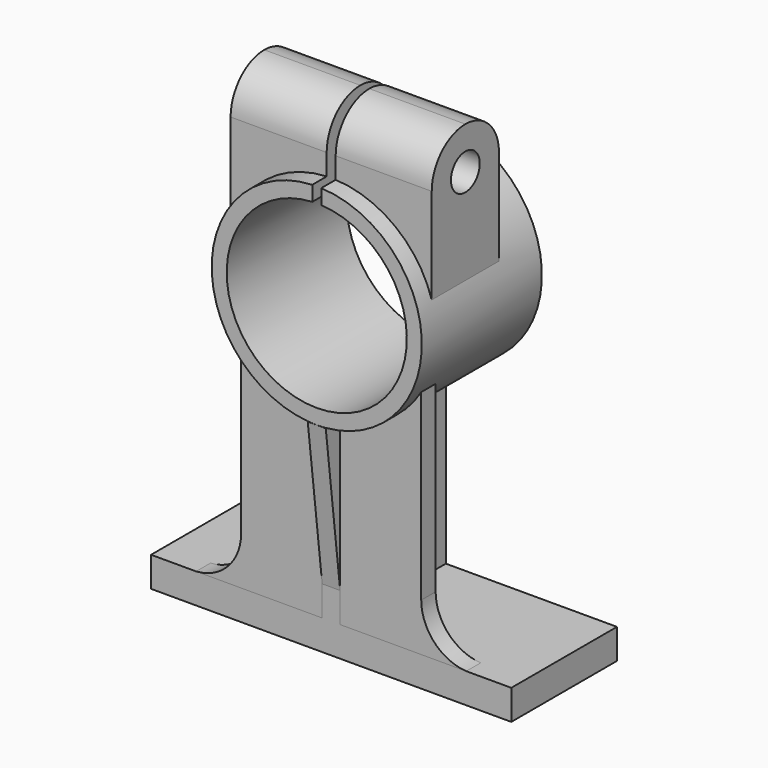
from build123d import *

# Parameters (mm, degrees)
F1_DEPTH = 6
F2_DEPTH = 44
F0_W     = 6
F0_H     = 10
F3_DEPTH = 6
F4_DEPTH = 28
F6_DEPTH = 93.501
F7_DEPTH = 93.501


with BuildPart() as f1:
    # F0 (on Front) → F1 (new body)
    with BuildSketch(Plane.XZ):
        with BuildLine():
            ThreePointArc((-33.5, 10.1365674664), (-34.7328343847, -4.3162733471), (-30, -18.0277563773))
            ThreePointArc((-30, -18.0277563773), (-18.5249919592, -29.695532878), (-3, -34.8711915483))
            ThreePointArc((-3, -34.8711915483), (-1.5013819904, -34.9677830598), (1.54e-08, -35))
            ThreePointArc((1.54e-08, -35), (1.5013820058, -34.9677830592), (3, -34.8711915483))
            ThreePointArc((3, -34.8711915483), (18.5249919592, -29.695532878), (30, -18.0277563773))
            ThreePointArc((30, -18.0277563773), (34.7328343847, -4.3162733471), (33.5, 10.1365674664))
            ThreePointArc((33.5, 10.1365674664), (21.4568882491, 27.6514366113), (1.5, 34.9678423698))
            Line((1.5, 34.9678423698), (1.5, 29.9624765332))
            ThreePointArc((1.5, 29.9624765332), (0, -30), (-1.5, 29.9624765332))
            Line((-1.5, 29.9624765332), (-1.5, 34.9678423698))
            ThreePointArc((-1.5, 34.9678423698), (-21.4568882491, 27.6514366113), (-33.5, 10.1365674664))
        make_face()
    extrude(amount=F1_DEPTH)

    # F0 (on Front) → F2 (join)
    with BuildSketch(Plane.XZ):
        with BuildLine():
            ThreePointArc((-33.5, 10.1365674664), (-34.7328343847, -4.3162733471), (-30, -18.0277563773))
            ThreePointArc((-30, -18.0277563773), (-18.5249919592, -29.695532878), (-3, -34.8711915483))
            ThreePointArc((-3, -34.8711915483), (-1.5013819904, -34.9677830598), (1.54e-08, -35))
            ThreePointArc((1.54e-08, -35), (1.5013820058, -34.9677830592), (3, -34.8711915483))
            ThreePointArc((3, -34.8711915483), (18.5249919592, -29.695532878), (30, -18.0277563773))
            ThreePointArc((30, -18.0277563773), (34.7328343847, -4.3162733471), (33.5, 10.1365674664))
            ThreePointArc((33.5, 10.1365674664), (21.4568882491, 27.6514366113), (1.5, 34.9678423698))
            Line((1.5, 34.9678423698), (1.5, 29.9624765332))
            ThreePointArc((1.5, 29.9624765332), (0, -30), (-1.5, 29.9624765332))
            Line((-1.5, 29.9624765332), (-1.5, 34.9678423698))
            ThreePointArc((-1.5, 34.9678423698), (-21.4568882491, 27.6514366113), (-33.5, 10.1365674664))
        make_face()
    extrude(amount=-F2_DEPTH)

    # F0 (on Front) → F3 (join)
    with BuildSketch(Plane.XZ):
        with BuildLine():
            Line((-30, -18.0277563773), (-30, -35))
            Line((-30, -35), (-3, -35))
            Line((-3, -35), (-3, -34.8711915483))
            ThreePointArc((-3, -34.8711915483), (-18.5249919592, -29.695532878), (-30, -18.0277563773))
        make_face()
        with BuildLine():
            Line((3, -34.8711915483), (3, -35))
            Line((3, -35), (30, -35))
            Line((30, -35), (30, -18.0277563773))
            ThreePointArc((30, -18.0277563773), (18.5249919592, -29.695532878), (3, -34.8711915483))
        make_face()
        with BuildLine():
            Line((-30, -95), (-30, -79.0312805773))
            ThreePointArc((-30, -79.0312805773), (-34.3380962103, -89.9857317274), (-45, -95))
            Line((-45, -95), (-30, -95))
        make_face()
        with BuildLine():
            ThreePointArc((45, -95), (34.3380962103, -89.9857317274), (30, -79.0312805773))
            Line((30, -79.0312805773), (30, -95))
            Line((30, -95), (45, -95))
        make_face()
        Polygon((-3, -35), (-30, -35), (-30, -79.0312805773), (-30, -95), (-3, -95), (-3, -85), align=None)
        Polygon((30, -35), (3, -35), (3, -85), (3, -95), (30, -95), (30, -79.0312805773), align=None)
    extrude(amount=-F3_DEPTH)

    # F0 (on Front) → F4 (join)
    with BuildSketch(Plane.XZ):
        with BuildLine():
            Line((-33.5, 56), (-33.5, 10.1365674664))
            ThreePointArc((-33.5, 10.1365674664), (-21.4568882491, 27.6514366113), (-1.5, 34.9678423698))
            Line((-1.5, 34.9678423698), (-1.5, 56))
            Line((-1.5, 56), (-33.5, 56))
        make_face()
        with BuildLine():
            ThreePointArc((1.5, 34.9678423698), (21.4568882491, 27.6514366113), (33.5, 10.1365674664))
            Line((33.5, 10.1365674664), (33.5, 56))
            Line((33.5, 56), (1.5, 56))
            Line((1.5, 56), (1.5, 34.9678423698))
        make_face()
    extrude(amount=-F4_DEPTH)


with BuildPart() as f1b:
    # F0 (on Front) → F1, piece 2 (new body)
    with BuildSketch(Plane.XZ):
        Polygon((1.54e-08, -35), (-3, -35), (-3, -85), (3, -85), (3, -35), align=None)
    extrude(amount=F1_DEPTH)

    # F0 (on Front) → F2, piece 2 (join)
    with BuildSketch(Plane.XZ):
        Polygon((1.54e-08, -35), (-3, -35), (-3, -85), (3, -85), (3, -35), align=None)
        Polygon((-3, -95), (-30, -95), (-45, -95), (-60, -95), (-60, -105), (60, -105), (60, -95), (45, -95), (30, -95), (3, -95), align=None)
        with Locations((0, -90)):
            Rectangle(F0_W, F0_H)
    extrude(amount=-F2_DEPTH)


with BuildPart() as f6_tool:
    # F5 (on face) → F6 (new body, through all)
    with BuildSketch(Plane(origin=(-33.5, 0, 0), x_dir=(0, -1, 0), z_dir=(-1, 0, 0))):
        with BuildLine():
            ThreePointArc((-28, 42), (-23.8994949366, 51.8994949366), (-14, 56))
            Line((-14, 56), (-28, 56))
            Line((-28, 56), (-28, 42))
        make_face()
        with BuildLine():
            ThreePointArc((-14, 56), (-4.1005050634, 51.8994949366), (0, 42))
            Line((0, 42), (0, 56))
            Line((0, 56), (-14, 56))
        make_face()
        with BuildLine():
            Line((-20, 42), (-8, 42))
            ThreePointArc((-8, 42), (-14, 48), (-20, 42))
        make_face()
        with BuildLine():
            ThreePointArc((-20, 42), (-14, 36), (-8, 42))
            Line((-8, 42), (-20, 42))
        make_face()
        Polygon((0, -85), (6, -85), (6, -35), align=None)
    extrude(amount=-F6_DEPTH)


with BuildPart() as f1_1:
    add(f1.part)

    # F6: cut by f6_tool
    add(f6_tool.part, mode=Mode.SUBTRACT)

    # F5 (on face) → F7 (cut, through all)
    with BuildSketch(Plane(origin=(-33.5, 0, 0), x_dir=(0, -1, 0), z_dir=(-1, 0, 0))):
        Polygon((0, -85), (6, -85), (6, -35), align=None)
    extrude(amount=-F7_DEPTH, mode=Mode.SUBTRACT)


with BuildPart() as f1b_1:
    add(f1b.part)

    # F6: cut by f6_tool
    add(f6_tool.part, mode=Mode.SUBTRACT)


solid = Compound([f1_1.part, f1b_1.part])
